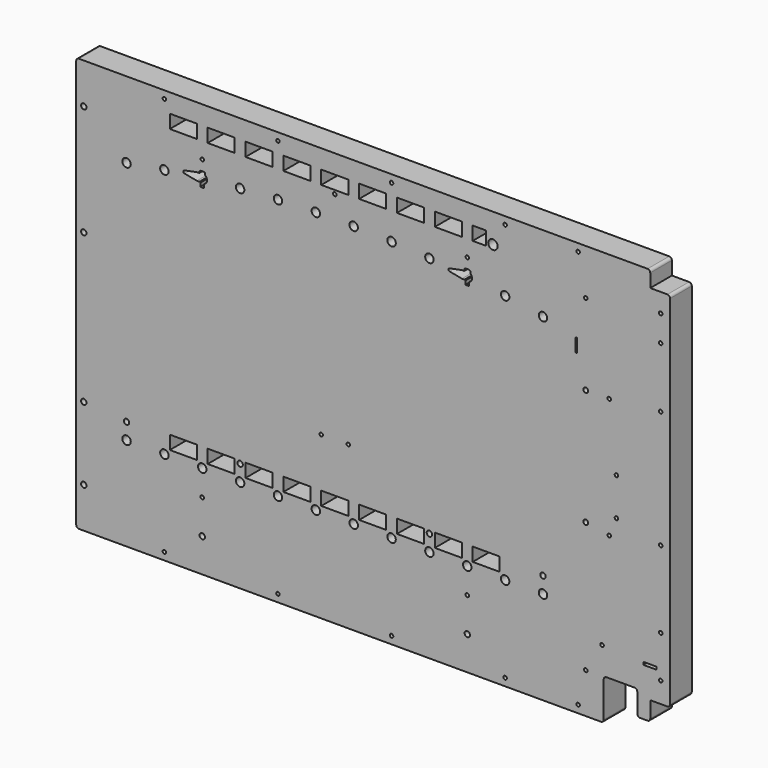
from build123d import *

# Parameters (mm, degrees)
F0_R     = 2.54
F0_R_2   = 1.651
F0_R_3   = 3.96875
F0_W     = 25.4
F0_H     = 12.7
F0_R_4   = 1.6637
F0_W_2   = 12.3180602
F0_H_2   = 2.54
F0_R_5   = 2.286
F0_R_6   = 4.445
F0_W_3   = 12.7
F0_W_4   = 1.6764
F1_DEPTH = 25.4


# Not quite as in the source:
# - ends of sketch curves that miss each other by under 0.0002 mm in the source are joined


with BuildPart() as f1:
    # F0 (on Front) → F1 (new body)
    with BuildSketch(Plane.XZ):
        with BuildLine():
            ThreePointArc((276.3642174, -154.0206978), (278.1602686242, -153.2767490242), (278.9042174, -151.4806978))
            Line((278.9042174, -151.4806978), (278.9042174, 184.2057022))
            ThreePointArc((278.9042174, 184.2057022), (278.1602686242, 186.0017534242), (276.3642174, 186.7457022))
            Line((276.3642174, 186.7457022), (260.2361572, 186.7457022))
            Line((260.2361572, 186.7457022), (260.2361572, 199.3177624))
            ThreePointArc((260.2361572, 199.3177624), (259.4922084242, 201.1138136242), (257.6961572, 201.8577624))
            Line((257.6961572, 201.8577624), (-276.3642428, 201.8577624))
            ThreePointArc((-276.3642428, 201.8577624), (-278.1602940242, 201.1138136242), (-278.9042428, 199.3177624))
            Line((-278.9042428, 199.3177624), (-278.9042428, -184.372758))
            ThreePointArc((-278.9042428, -184.372758), (-278.1602940242, -186.1688092242), (-276.3642428, -186.912758))
            Line((-276.3642428, -186.912758), (214.0081572, -186.912758))
            ThreePointArc((214.0081572, -186.912758), (215.8042084242, -186.1688092242), (216.5481572, -184.372758))
            Line((216.5481572, -184.372758), (216.5481572, -150.9726978))
            ThreePointArc((216.5481572, -150.9726978), (217.2921059758, -149.1766465758), (219.0881572, -148.4326978))
            Line((219.0881572, -148.4326978), (245.5041572, -148.4326978))
            ThreePointArc((245.5041572, -148.4326978), (247.3002084242, -149.1766465758), (248.0441572, -150.9726978))
            Line((248.0441572, -150.9726978), (248.0441572, -169.2606978))
            ThreePointArc((248.0441572, -169.2606978), (248.7881059758, -171.0567490242), (250.5841572, -171.8006978))
            Line((250.5841572, -171.8006978), (257.6961572, -171.8006978))
            ThreePointArc((257.6961572, -171.8006978), (259.4922084242, -171.0567490242), (260.2361572, -169.2606978))
            Line((260.2361572, -169.2606978), (260.2361572, -154.0206978))
            Line((260.2361572, -154.0206978), (276.3642174, -154.0206978))
        make_face()
        with Locations((-271.7922428, -148.9406978)):
            Circle(F0_R, mode=Mode.SUBTRACT)
        with Locations((-196.1002428, -179.800758)):
            Circle(F0_R_2, mode=Mode.SUBTRACT)
        with Locations((-160.5402428, -155.2906978)):
            Circle(F0_R, mode=Mode.SUBTRACT)
        with Locations((-231.6602428, -99.0042978)):
            Circle(F0_R_3, mode=Mode.SUBTRACT)
        with Locations((-160.5402428, -123.1342978)):
            Circle(F0_R_2, mode=Mode.SUBTRACT)
        with Locations((-196.1002428, -99.0042978)):
            Circle(F0_R_3, mode=Mode.SUBTRACT)
        with Locations((-160.5402428, -99.0042978)):
            Circle(F0_R_3, mode=Mode.SUBTRACT)
        with Locations((-89.4202428, -179.800758)):
            Circle(F0_R_2, mode=Mode.SUBTRACT)
        with Locations((-124.9802428, -99.0042978)):
            Circle(F0_R_3, mode=Mode.SUBTRACT)
        with Locations((-89.4202428, -99.0042978)):
            Circle(F0_R_3, mode=Mode.SUBTRACT)
        with Locations((-53.8602428, -99.0042978)):
            Circle(F0_R_3, mode=Mode.SUBTRACT)
        with Locations((-18.3002428, -99.0042978)):
            Circle(F0_R_3, mode=Mode.SUBTRACT)
        with Locations((-271.7922428, -80.3606978)):
            Circle(F0_R, mode=Mode.SUBTRACT)
        with Locations((-231.6602428, -83.7642978)):
            Circle(F0_R, mode=Mode.SUBTRACT)
        with Locations((-178.3202428, -87.5742978)):
            Rectangle(F0_W, F0_H, mode=Mode.SUBTRACT)
        with Locations((-142.7602428, -87.5742978)):
            Rectangle(F0_W, F0_H, mode=Mode.SUBTRACT)
        with Locations((-124.9802428, -83.7642978)):
            Circle(F0_R, mode=Mode.SUBTRACT)
        with Locations((-107.2002428, -87.5742978)):
            Rectangle(F0_W, F0_H, mode=Mode.SUBTRACT)
        with Locations((-71.6402428, -87.5742978)):
            Rectangle(F0_W, F0_H, mode=Mode.SUBTRACT)
        with Locations((-36.0802428, -87.5742978)):
            Rectangle(F0_W, F0_H, mode=Mode.SUBTRACT)
        with Locations((-0.5202428, -87.5742978)):
            Rectangle(F0_W, F0_H, mode=Mode.SUBTRACT)
        with Locations((-48.7802428, -34.8692978)):
            Circle(F0_R_2, mode=Mode.SUBTRACT)
        with Locations((-23.3802428, -34.8692978)):
            Circle(F0_R_2, mode=Mode.SUBTRACT)
        with Locations((17.2597572, -179.800758)):
            Circle(F0_R_2, mode=Mode.SUBTRACT)
        with Locations((123.9397572, -179.800758)):
            Circle(F0_R_2, mode=Mode.SUBTRACT)
        with Locations((88.3797572, -155.2906978)):
            Circle(F0_R, mode=Mode.SUBTRACT)
        with Locations((17.2597572, -99.0042978)):
            Circle(F0_R_3, mode=Mode.SUBTRACT)
        with Locations((52.8197572, -99.0042978)):
            Circle(F0_R_3, mode=Mode.SUBTRACT)
        with Locations((88.3797572, -123.1342978)):
            Circle(F0_R_2, mode=Mode.SUBTRACT)
        with Locations((88.3797572, -99.0042978)):
            Circle(F0_R_3, mode=Mode.SUBTRACT)
        with Locations((123.9397572, -99.0042978)):
            Circle(F0_R_3, mode=Mode.SUBTRACT)
        with Locations((192.5197572, -179.800758)):
            Circle(F0_R_2, mode=Mode.SUBTRACT)
        with Locations((199.6317572, -148.9406978)):
            Circle(F0_R_4, mode=Mode.SUBTRACT)
        with Locations((159.4997572, -99.0042978)):
            Circle(F0_R_3, mode=Mode.SUBTRACT)
        with Locations((214.9733572, -123.1342978)):
            Circle(F0_R_2, mode=Mode.SUBTRACT)
        with Locations((270.0142174, -134.5642978)):
            Circle(F0_R_2, mode=Mode.SUBTRACT)
        with Locations((260.0451873, -125.6742978)):
            Rectangle(F0_W_2, F0_H_2, mode=Mode.SUBTRACT)
        with Locations((270.0142174, -95.1942978)):
            Circle(F0_R_2, mode=Mode.SUBTRACT)
        with Locations((35.0397572, -87.5742978)):
            Rectangle(F0_W, F0_H, mode=Mode.SUBTRACT)
        with Locations((52.8197572, -83.7642978)):
            Circle(F0_R, mode=Mode.SUBTRACT)
        with Locations((70.5997572, -87.5742978)):
            Rectangle(F0_W, F0_H, mode=Mode.SUBTRACT)
        with Locations((106.1597572, -87.5742978)):
            Rectangle(F0_W, F0_H, mode=Mode.SUBTRACT)
        with Locations((159.4997572, -83.7642978)):
            Circle(F0_R, mode=Mode.SUBTRACT)
        with Locations((199.6317572, -26.6142978)):
            Circle(F0_R_5, mode=Mode.SUBTRACT)
        with Locations((221.7297572, -30.4242978)):
            Circle(F0_R_4, mode=Mode.SUBTRACT)
        with Locations((270.0142174, -22.8042978)):
            Circle(F0_R_2, mode=Mode.SUBTRACT)
        with Locations((228.4861572, -13.9142978)):
            Circle(F0_R_4, mode=Mode.SUBTRACT)
        with Locations((-271.7922428, 59.7457022)):
            Circle(F0_R, mode=Mode.SUBTRACT)
        with Locations((-231.6602428, 130.3261554)):
            Circle(F0_R_3, mode=Mode.SUBTRACT)
        with Locations((-196.1002428, 135.9911174)):
            Circle(F0_R_3, mode=Mode.SUBTRACT)
        with BuildLine():
            Line((-163.3342428, 144.058513), (-163.3342428, 145.9205108))
            ThreePointArc((-163.3342428, 145.9205108), (-160.5402428, 146.598513), (-157.7462397986, 145.9205166202))
            Line((-157.7462397986, 145.9205166202), (-157.7462428, 143.9596308))
            ThreePointArc((-157.7462428, 143.9596308), (-156.1351486502, 139.9082314746), (-158.7622414095, 136.428603814))
            Line((-158.7622414095, 136.428603814), (-158.7622428, 133.0928504))
            ThreePointArc((-158.7622428, 133.0928504), (-160.5402428, 132.882513), (-162.3182430473, 133.0928493693))
            Line((-162.3182430473, 133.0928493693), (-162.3182428, 136.428607))
            ThreePointArc((-162.3182428, 136.428607), (-162.7777786816, 136.6617502921), (-163.2072428, 136.946513))
            Line((-163.2072428, 136.946513), (-165.6202428, 136.946513))
            Line((-165.6202428, 136.946513), (-177.2967244, 139.2566684))
            ThreePointArc((-177.2967244, 139.2566684), (-178.3202428, 140.502513), (-177.2967257795, 141.7483645726))
            Line((-177.2967257795, 141.7483645726), (-165.6202428, 144.058513))
            Line((-165.6202428, 144.058513), (-163.3342428, 144.058513))
        make_face(mode=Mode.SUBTRACT)
        with Locations((-271.7922428, 163.8857022)):
            Circle(F0_R, mode=Mode.SUBTRACT)
        with Locations((-160.5402428, 156.2657022)):
            Circle(F0_R_2, mode=Mode.SUBTRACT)
        with Locations((-178.3202428, 177.8557022)):
            Rectangle(F0_W, F0_H, mode=Mode.SUBTRACT)
        with Locations((-196.1002428, 194.7457624)):
            Circle(F0_R_2, mode=Mode.SUBTRACT)
        with Locations((-142.7602428, 177.8557022)):
            Rectangle(F0_W, F0_H, mode=Mode.SUBTRACT)
        with Locations((-124.9802428, 143.8742106)):
            Circle(F0_R_3, mode=Mode.SUBTRACT)
        with Locations((-89.4202428, 146.116421)):
            Circle(F0_R_3, mode=Mode.SUBTRACT)
        with Locations((-53.8602428, 147.2358498)):
            Circle(F0_R_3, mode=Mode.SUBTRACT)
        with Locations((-18.3002428, 147.2358498)):
            Circle(F0_R_3, mode=Mode.SUBTRACT)
        with Locations((-107.2002428, 177.8557022)):
            Rectangle(F0_W, F0_H, mode=Mode.SUBTRACT)
        with Locations((-71.6402428, 177.8557022)):
            Rectangle(F0_W, F0_H, mode=Mode.SUBTRACT)
        with Locations((-89.4202428, 194.7457624)):
            Circle(F0_R_2, mode=Mode.SUBTRACT)
        with Locations((-36.0802428, 167.9497022)):
            Circle(F0_R_2, mode=Mode.SUBTRACT)
        with Locations((-36.0802428, 177.8557022)):
            Rectangle(F0_W, F0_H, mode=Mode.SUBTRACT)
        with Locations((-0.5202428, 177.8557022)):
            Rectangle(F0_W, F0_H, mode=Mode.SUBTRACT)
        with Locations((228.4861572, 21.6457022)):
            Circle(F0_R_4, mode=Mode.SUBTRACT)
        with Locations((199.6317572, 82.6057022)):
            Circle(F0_R_5, mode=Mode.SUBTRACT)
        with Locations((221.7297572, 82.6057022)):
            Circle(F0_R_4, mode=Mode.SUBTRACT)
        with Locations((270.0142174, 87.6857022)):
            Circle(F0_R_2, mode=Mode.SUBTRACT)
        with Locations((17.2597572, 146.116421)):
            Circle(F0_R_3, mode=Mode.SUBTRACT)
        with Locations((52.8197572, 143.8742106)):
            Circle(F0_R_3, mode=Mode.SUBTRACT)
        with BuildLine():
            Line((85.5857572, 144.058513), (85.5857572, 145.9205108))
            ThreePointArc((85.5857572, 145.9205108), (88.3797572, 146.598513), (91.1737602014, 145.9205166202))
            Line((91.1737602014, 145.9205166202), (91.1737572, 143.9596308))
            ThreePointArc((91.1737572, 143.9596308), (92.7848513498, 139.9082314746), (90.1577585905, 136.428603814))
            Line((90.1577585905, 136.428603814), (90.1577572, 133.0928504))
            ThreePointArc((90.1577572, 133.0928504), (88.3797572, 132.882513), (86.6017569527, 133.0928493693))
            Line((86.6017569527, 133.0928493693), (86.6017572, 136.428607))
            ThreePointArc((86.6017572, 136.428607), (86.1422213184, 136.6617502921), (85.7127572, 136.946513))
            Line((85.7127572, 136.946513), (83.2997572, 136.946513))
            Line((83.2997572, 136.946513), (71.6232756, 139.2566684))
            ThreePointArc((71.6232756, 139.2566684), (70.5997572, 140.502513), (71.6232742205, 141.7483645726))
            Line((71.6232742205, 141.7483645726), (83.2997572, 144.058513))
            Line((83.2997572, 144.058513), (85.5857572, 144.058513))
        make_face(mode=Mode.SUBTRACT)
        with Locations((123.9397572, 135.9911174)):
            Circle(F0_R_3, mode=Mode.SUBTRACT)
        with Locations((17.2597572, 194.7457624)):
            Circle(F0_R_2, mode=Mode.SUBTRACT)
        with Locations((35.0397572, 177.8557022)):
            Rectangle(F0_W, F0_H, mode=Mode.SUBTRACT)
        with Locations((88.3797572, 156.2657022)):
            Circle(F0_R_2, mode=Mode.SUBTRACT)
        with Locations((112.5097572, 174.6045022)):
            Circle(F0_R_6, mode=Mode.SUBTRACT)
        with Locations((70.5997572, 177.8557022)):
            Rectangle(F0_W, F0_H, mode=Mode.SUBTRACT)
        with Locations((99.8097572, 177.8557022)):
            Rectangle(F0_W_3, F0_H, mode=Mode.SUBTRACT)
        with Locations((123.9397572, 194.7457624)):
            Circle(F0_R_2, mode=Mode.SUBTRACT)
        with Locations((190.787274, 116.8957022)):
            Rectangle(F0_W_4, F0_H, mode=Mode.SUBTRACT)
        with Locations((159.4997572, 130.3261554)):
            Circle(F0_R_3, mode=Mode.SUBTRACT)
        with Locations((270.0142174, 144.3531022)):
            Circle(F0_R_2, mode=Mode.SUBTRACT)
        with Locations((199.6317572, 158.8057022)):
            Circle(F0_R_4, mode=Mode.SUBTRACT)
        with Locations((192.5197572, 194.7457624)):
            Circle(F0_R_2, mode=Mode.SUBTRACT)
        with Locations((270.0142174, 168.9657022)):
            Circle(F0_R_2, mode=Mode.SUBTRACT)
    extrude(amount=F1_DEPTH)


solid = f1.part
